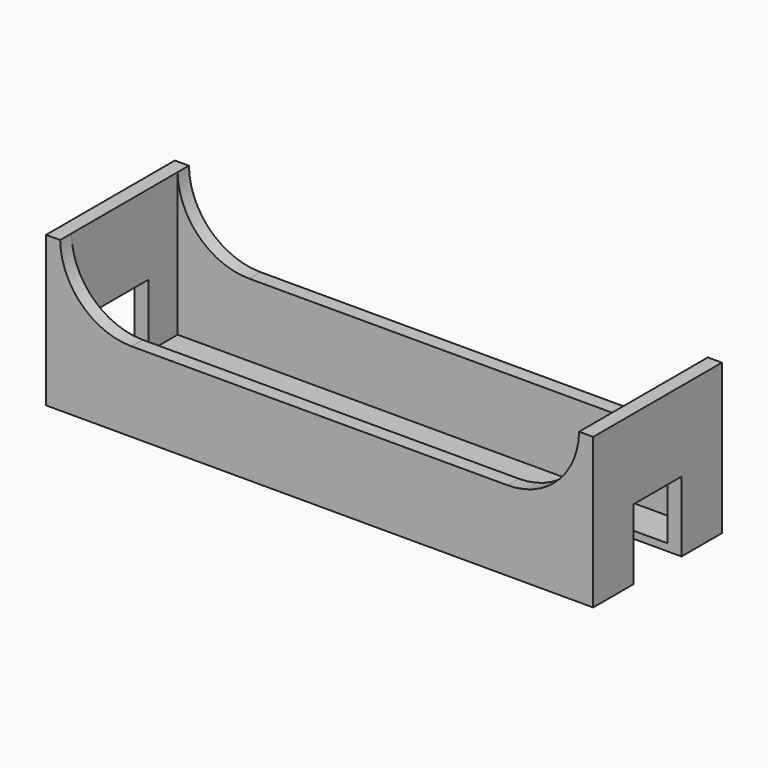
from build123d import *

# Parameters (mm, degrees)
F0_W          = 77.724
F0_H          = 22.86
F1_DEPTH      = 21.336
F2_W          = 73.724
F2_H          = 18.86
F3_DEPTH      = 20.32
F4_W          = 7.62
F4_H          = 8.5
F5_DEPTH      = 10
F6_W          = 73.724
F6_H          = 10
F7_DEPTH      = 25
F7_DEPTH_BACK = 25
F8_T1_DEPTH   = 2
F8_T3_DEPTH   = 2
F8_T8_DEPTH   = 52.7937003968
F8_T14_DEPTH  = 52.7937003968
F8_T20_DEPTH  = 52.7937003968
F8_T26_DEPTH  = 52.7937003968


# Not quite as in the source:
# - a fillet or chamfer that OpenCascade refuses, or shapes differently, is made with other operations: its cross-section is extruded or revolved along the edge and cut away or added


with BuildPart() as f1:
    # F0 (on Top) → F1 (new body)
    with BuildSketch(Plane.XY):
        with Locations((38.862, 11.43)):
            Rectangle(F0_W, F0_H)
    extrude(amount=F1_DEPTH)

    # F2 (on face) → F3 (cut)
    with BuildSketch(Plane.XY.offset(21.336)):
        with Locations((38.862, 11.43)):
            Rectangle(F2_W, F2_H)
    extrude(amount=-F3_DEPTH, mode=Mode.SUBTRACT)

    # F4 (on face) → F5 (cut)
    with BuildSketch(Plane(origin=(0, 0, 0), x_dir=(1, 0, 0), z_dir=(0, 0, -1))):
        with Locations((3.81, -11.43)):
            Rectangle(F4_W, F4_H)
        with Locations((73.914, -11.43)):
            Rectangle(F4_W, F4_H)
    extrude(amount=-F5_DEPTH, mode=Mode.SUBTRACT)

    # F6 (on Front) → F7 (cut, two sides)
    with BuildSketch(Plane.XZ) as f7_sk:
        with Locations((38.862, 16.336)):
            Rectangle(F6_W, F6_H)
    extrude(amount=-F7_DEPTH, mode=Mode.SUBTRACT)
    extrude(f7_sk.sketch, amount=F7_DEPTH_BACK, mode=Mode.SUBTRACT)

    # F8: fillet of radius 10.16 on 4 edges, made by hand

    # F8_s2 → F8_t1 (join)
    with BuildSketch(Plane.XZ.offset(-2)):
        with BuildLine():
            ThreePointArc((12.1587400794, 11.336), (5.0313282069, 14.2554475349), (2, 21.336))
            Line((2, 21.336), (2, 11.336))
            Line((2, 11.336), (12.1587400794, 11.336))
        make_face()
        with BuildLine():
            ThreePointArc((65.5652599206, 11.336), (72.6926717931, 14.2554475349), (75.724, 21.336))
            Line((75.724, 21.336), (75.724, 11.336))
            Line((75.724, 11.336), (65.5652599206, 11.336))
        make_face()
    extrude(amount=F8_T1_DEPTH)

    # F8_s4 → F8_t3 (join)
    with BuildSketch(Plane.XZ.offset(-22.86)):
        with BuildLine():
            ThreePointArc((12.1587400794, 11.336), (5.0313282069, 14.2554475349), (2, 21.336))
            Line((2, 21.336), (2, 11.336))
            Line((2, 11.336), (12.1587400794, 11.336))
        make_face()
        with BuildLine():
            ThreePointArc((75.724, 21.336), (72.6926717931, 14.2554475349), (65.5652599206, 11.336))
            Line((65.5652599206, 11.336), (75.724, 11.336))
            Line((75.724, 11.336), (75.724, 21.336))
        make_face()
    extrude(amount=F8_T3_DEPTH)


with BuildPart() as f8_tool6:
    # F8_s7 → F8_t8 (new body)
    with BuildSketch(Plane.XZ.offset(-27.3968501984)):
        with BuildLine():
            ThreePointArc((12.1587400794, 11.336), (5.0313282069, 14.2554475349), (2, 21.336))
            Line((2, 21.336), (2, 11.336))
            Line((2, 11.336), (12.1587400794, 11.336))
        make_face()
    extrude(amount=F8_T8_DEPTH)

    split(bisect_by=Plane.XZ.offset(-22.86), keep=Keep.TOP)

    split(bisect_by=Plane.XZ.offset(-20.86), keep=Keep.BOTTOM)


with BuildPart() as f1_1:
    add(f1.part)

    # F8_t5: union F8_tool6
    add(f8_tool6.part)


with BuildPart() as f8_tool12:
    # F8_s13 → F8_t14 (new body)
    with BuildSketch(Plane.XZ.offset(-48.2568501984)):
        with BuildLine():
            ThreePointArc((12.1587400794, 11.336), (5.0313282069, 14.2554475349), (2, 21.336))
            Line((2, 21.336), (2, 11.336))
            Line((2, 11.336), (12.1587400794, 11.336))
        make_face()
    extrude(amount=F8_T14_DEPTH)

    split(bisect_by=Plane.XZ.offset(-2), keep=Keep.TOP)

    split(bisect_by=Plane.XZ, keep=Keep.BOTTOM)


with BuildPart() as f1_2:
    add(f1_1.part)

    # F8_t11: union F8_tool12
    add(f8_tool12.part)


with BuildPart() as f8_tool18:
    # F8_s19 → F8_t20 (new body)
    with BuildSketch(Plane.XZ.offset(25.3968501984)):
        with BuildLine():
            ThreePointArc((65.5652599206, 11.336), (72.6926717931, 14.2554475349), (75.724, 21.336))
            Line((75.724, 21.336), (75.724, 11.336))
            Line((75.724, 11.336), (65.5652599206, 11.336))
        make_face()
    extrude(amount=-F8_T20_DEPTH)

    split(bisect_by=Plane.XZ.offset(-22.86), keep=Keep.TOP)

    split(bisect_by=Plane.XZ.offset(-20.86), keep=Keep.BOTTOM)


with BuildPart() as f1_3:
    add(f1_2.part)

    # F8_t17: union F8_tool18
    add(f8_tool18.part)


with BuildPart() as f8_tool24:
    # F8_s25 → F8_t26 (new body)
    with BuildSketch(Plane.XZ.offset(4.5368501984)):
        with BuildLine():
            ThreePointArc((75.724, 21.336), (72.6926717931, 14.2554475349), (65.5652599206, 11.336))
            Line((65.5652599206, 11.336), (75.724, 11.336))
            Line((75.724, 11.336), (75.724, 21.336))
        make_face()
    extrude(amount=-F8_T26_DEPTH)

    split(bisect_by=Plane.XZ.offset(-2), keep=Keep.TOP)

    split(bisect_by=Plane.XZ, keep=Keep.BOTTOM)


with BuildPart() as f1_4:
    add(f1_3.part)

    # F8_t23: union F8_tool24
    add(f8_tool24.part)


solid = f1_4.part
